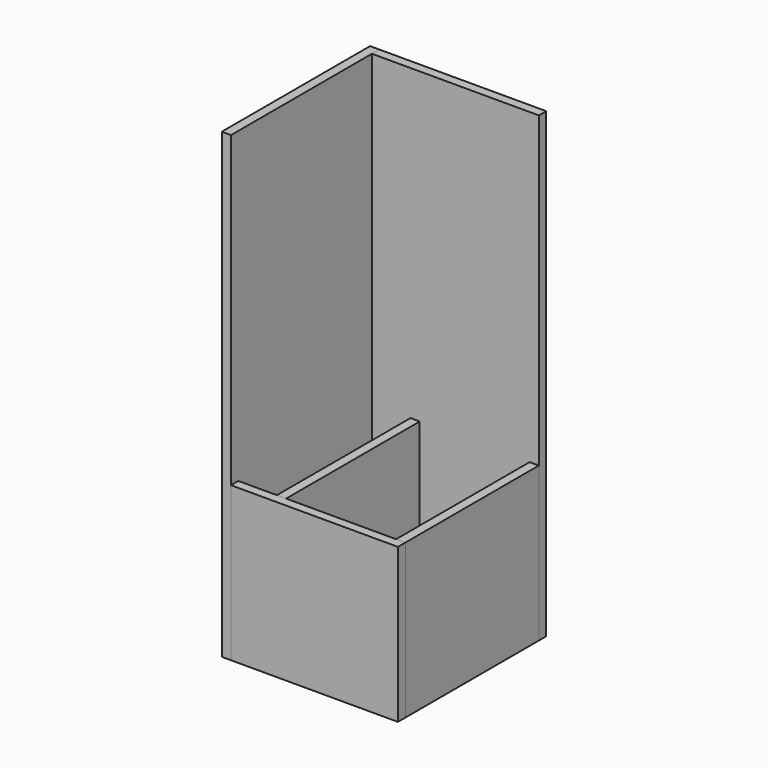
from build123d import *

# Parameters (mm, degrees)
F4_W      = 311.94375
F4_H      = 330.2
F5_DEPTH  = 18.25625
F6_DEPTH  = 914.4
F7_DEPTH  = 914.4
F8_DEPTH  = 304.8
F3_W      = 18.25625
F3_H      = 330.2
F9_DEPTH  = 304.8
F10_W     = 18.25625
F10_H     = 330.2
F11_DEPTH = 286.54375


# Not quite as in the source:
# - a length typed as a fraction of an inch, garbled in the dataset ("3 / 203.2 mm" for 3/8 in), is restored


with BuildPart() as f5:
    # F4 (on Top) → F5 (new body)
    with BuildSketch(Plane.XY):
        Rectangle(F4_W, F4_H)
    extrude(amount=F5_DEPTH)


with BuildPart() as f6:
    # F3 (on Top) → F6 (new body)
    with BuildSketch(Plane.XY):
        Polygon((-174.228125, -183.35625), (-155.971875, -183.35625), (-155.971875, -165.1), (-155.971875, 165.1), (-155.971875, 183.35625), (-174.228125, 183.35625), align=None)
    extrude(amount=F6_DEPTH)


with BuildPart() as f7:
    # F3 (on Top) → F7 (new body)
    with BuildSketch(Plane.XY):
        Polygon((155.971875, 165.1), (174.228125, 165.1), (174.228125, 183.35625), (-155.971875, 183.35625), (-155.971875, 165.1), align=None)
    extrude(amount=F7_DEPTH)


with BuildPart() as f8:
    # F3 (on Top) → F8 (new body)
    with BuildSketch(Plane.XY):
        Polygon((-155.971875, -183.35625), (174.228125, -183.35625), (174.228125, -165.1), (155.971875, -165.1), (-155.971875, -165.1), align=None)
    extrude(amount=F8_DEPTH)


with BuildPart() as f9:
    # F3 (on Top) → F9 (new body)
    with BuildSketch(Plane.XY):
        with Locations((165.1, 0)):
            Rectangle(F3_W, F3_H)
    extrude(amount=F9_DEPTH)


with BuildPart() as f11:
    # F10 (on face) → F11 (new body, through all)
    with BuildSketch(Plane.XY.offset(18.25625)):
        with Locations((-70.64375, 0)):
            Rectangle(F10_W, F10_H)
    extrude(amount=F11_DEPTH)


solid = Compound([f5.part, f6.part, f7.part, f8.part, f9.part, f11.part])
